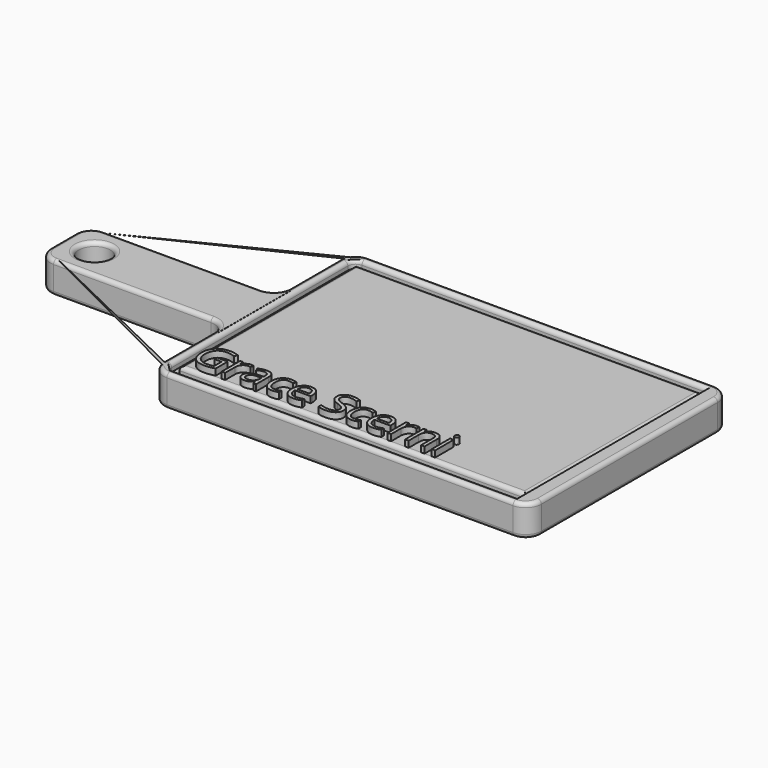
from build123d import *

# Parameters (mm, degrees)
F0_W         = 152.4
F0_H         = 50.8
F1_DEPTH     = 25.4
F2_R         = 12.7
F3_DEPTH     = 25.4
F5_DEPTH     = 6.35
F6_R         = 6.35
F7_R         = 12.7
F8_R         = 3.17499
F9_TEXT_SIZE = 34.8112854007
F10_DEPTH    = 5.08


# Not quite as in the source:
# - a fillet or chamfer is up to 0.001 mm smaller than in the source, because OpenCascade refuses the exact size
# - Text() gives the source's letters only with a copy of the font that has no kerning and outlines rounded to 1/6400 em; it was checked with that copy


with BuildPart() as f1:
    # F0 (on Top) → F1 (new body)
    with BuildSketch(Plane.XY):
        Polygon((0, 76.2), (0, 0), (304.8, 0), (304.8, 203.2), (0, 203.2), (0, 127), align=None)
        with Locations((-76.2, 101.6)):
            Rectangle(F0_W, F0_H)
    extrude(amount=F1_DEPTH)

    # F2 (on face) → F3 (cut)
    with BuildSketch(Plane.XY.offset(25.4)):
        with Locations((-127, 101.6)):
            Circle(F2_R)
    extrude(amount=-F3_DEPTH, mode=Mode.SUBTRACT)

    # F4 (on face) → F5 (cut)
    with BuildSketch(Plane.XY.offset(25.4)):
        Polygon((298.45, 196.85), (6.35, 196.85), (6.35, 127), (6.35, 76.2), (6.35, 6.35), (298.45, 6.35), align=None)
        Polygon((12.7, 76.2), (12.7, 127), (12.7, 190.5), (292.1, 190.5), (292.1, 12.7), (12.7, 12.7), align=None, mode=Mode.SUBTRACT)
    extrude(amount=-F5_DEPTH, mode=Mode.SUBTRACT)

    # F6
    f6_edges = [f1.edges().sort_by_distance(p)[0] for p in [
        (6.35, 196.85, 22.225),
        (298.45, 196.85, 22.225),
        (298.45, 6.35, 22.225),
        (6.35, 6.35, 22.225),
    ]]
    fillet(f6_edges, radius=F6_R)

    # F7
    f7_edges = [f1.edges().sort_by_distance(p)[0] for p in [
        (0, 0, 12.7),
        (304.8, 0, 12.7),
        (304.8, 203.2, 12.7),
        (0, 203.2, 12.7),
        (0, 127, 12.7),
        (0, 76.2, 12.7),
        (-152.4, 76.2, 12.7),
        (-152.4, 127, 12.7),
    ]]
    fillet(f7_edges, radius=F7_R)

    # F8 (radius 3.175 in the source; OpenCascade refuses exactly that, so slightly less here)
    f8_edges = [f1.edges().sort_by_distance(p)[0] for p in [
        (152.4, 190.5, 25.4),
        (292.1, 101.6, 25.4),
        (152.4, 12.7, 25.4),
        (12.7, 101.6, 25.4),
        (0, 38.1, 25.4),
        (-3.719744, 72.480256, 25.4),
        (3.719744, 3.719744, 25.4),
        (-76.2, 76.2, 25.4),
        (152.4, 0, 25.4),
        (-148.680256, 79.919744, 25.4),
        (301.080256, 3.719744, 25.4),
        (-152.4, 101.6, 25.4),
        (304.8, 101.6, 25.4),
        (-148.680256, 123.280256, 25.4),
        (301.080256, 199.480256, 25.4),
        (-76.2, 127, 25.4),
        (152.4, 203.2, 25.4),
        (-3.719744, 130.719744, 25.4),
        (3.719744, 199.480256, 25.4),
        (0, 165.1, 25.4),
        (152.4, 196.85, 25.4),
        (296.590128, 194.990128, 25.4),
        (8.209872, 194.990128, 25.4),
        (298.45, 101.6, 25.4),
        (6.35, 101.6, 25.4),
        (296.590128, 8.209872, 25.4),
        (8.209872, 8.209872, 25.4),
        (152.4, 6.35, 25.4),
        (-139.7, 101.6, 25.4),
        (0, 38.1, 0),
        (-3.719744, 72.480256, 0),
        (3.719744, 3.719744, 0),
        (-76.2, 76.2, 0),
        (152.4, 0, 0),
        (-148.680256, 79.919744, 0),
        (301.080256, 3.719744, 0),
        (-152.4, 101.6, 0),
        (304.8, 101.6, 0),
        (-148.680256, 123.280256, 0),
        (301.080256, 199.480256, 0),
        (-76.2, 127, 0),
        (152.4, 203.2, 0),
        (-3.719744, 130.719744, 0),
        (3.719744, 199.480256, 0),
        (0, 165.1, 0),
        (-139.7, 101.6, 0),
    ]]
    fillet(f8_edges, radius=F8_R)

    # F9 (on face) → F10 (join)
    with BuildSketch(Plane.XY.offset(25.4)):
        with Locations((15.875, 15.875)):
            Text('Grace Scerni', F9_TEXT_SIZE, font='Open Sans', text_align=(TextAlign.LEFT, TextAlign.BOTTOM))
    extrude(amount=F10_DEPTH)


solid = f1.part
